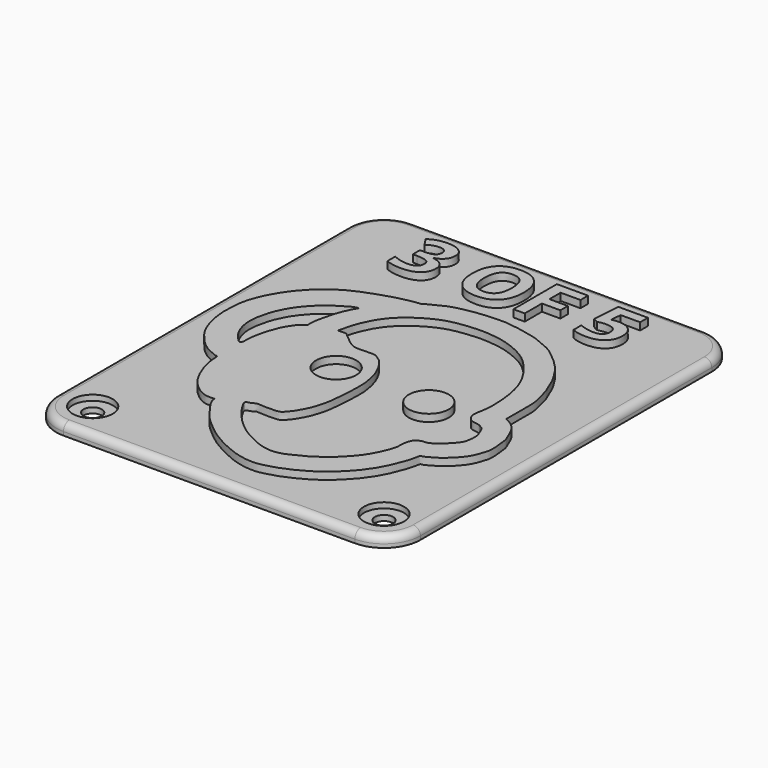
from build123d import *

# Parameters (mm, degrees)
F1_DEPTH     = 3
F2_R         = 5.5
F3_DEPTH     = 2
F4_R         = 2.5
F5_DEPTH     = 25
F4_R_2       = 5.5
F6_DEPTH     = 1.5
F7_R         = 2
F8_TEXT_SIZE = 20.8952981565
F9_DEPTH     = 2


# Not quite as in the source:
# - Text() gives the source's letters only with a copy of the font that has no kerning and outlines rounded to 1/6400 em; it was checked with that copy


with BuildPart() as f1:
    # F0 (on Top) → F1 (new body)
    with BuildSketch(Plane.XY):
        with BuildLine():
            Line((33.4852860868, 69.3044555187), (-46.5147139132, 69.3044555187))
            ThreePointArc((-46.5147139132, 69.3044555187), (-53.5857817251, 66.3755233306), (-56.5147139132, 59.3044555187))
            Line((-56.5147139132, 59.3044555187), (-56.5147139132, -40.6955444813))
            ThreePointArc((-56.5147139132, -40.6955444813), (-53.5857817251, -47.7666122931), (-46.5147139132, -50.6955444813))
            Line((-46.5147139132, -50.6955444813), (33.4852860868, -50.6955444813))
            ThreePointArc((33.4852860868, -50.6955444813), (40.5563538987, -47.7666122931), (43.4852860868, -40.6955444813))
            Line((43.4852860868, -40.6955444813), (43.4852860868, 59.3044555187))
            ThreePointArc((43.4852860868, 59.3044555187), (40.5563538987, 66.3755233306), (33.4852860868, 69.3044555187))
        make_face()
    extrude(amount=F1_DEPTH)

    # F2 (on face) → F3 (join)
    with BuildSketch(Plane.XY.offset(3)):
        with BuildLine():
            add(Edge.make_bspline(
                [(-18.6191648245, 37.6610159874), (-18.4103942017, 37.9016258723), (-16.7790980702, 38.6372652046), (-14.6637753752, 39.7765316628), (-13.2970537087, 40.3520065207), (-11.234009202, 40.9420295945), (-9.6324726991, 41.1696781496), (-8.0391436993, 41.5335651558), (-6.0169121605, 41.8153047571), (-4.3207068367, 41.9873935063), (-2.6143961302, 42.0419440702), (-0.9525336366, 42.1080518392), (1.0128601269, 42.1231970345), (2.1202521733, 41.9213075242), (4.0719475632, 41.6824185547), (5.8543562337, 41.3447673853), (8.2763433889, 40.8035747337), (10.1635651747, 40.353915966), (11.9937518037, 39.6067163832), (14.0226197173, 38.7871278462), (16.1856661814, 37.6734030141), (17.4924246856, 36.4788381138), (19.1253564081, 35.2746713919), (21.0525205789, 33.4368660129), (22.8143980711, 31.4334361407), (24.0610529234, 29.4392438038), (25.4962702164, 27.1113130015), (26.1960706131, 25.0093099567), (27.3364408686, 22.7329766681), (27.8343641487, 20.4595553566), (28.4512270226, 18.3747773676), (28.8543109039, 16.0260319825), (28.7482942364, 13.514319679), (28.7338146771, 10.334995111), (28.8639216748, 7.7618210354), (28.5892188921, 7.1456188181), (29.918494696, 6.6371361349), (30.7415769345, 6.048857602), (31.8218108898, 5.2284950474), (32.4881411718, 4.3144331607), (33.1106903749, 3.3497479147), (33.6641407706, 2.0109945661), (34.2180897974, 0.7680229197), (34.7699235136, -0.4925214664), (34.8393823017, -2.1248020855), (35.1159528786, -3.5786376005), (35.1890831283, -4.9707061488), (35.1986725747, -6.4306388091), (34.8113632413, -7.8018002545), (34.3648549572, -9.1685585465), (33.7006462016, -10.7925444113), (32.4786558474, -12.4867800792), (31.2093037355, -13.8794324624), (29.8228294921, -15.1123456384), (28.4481064283, -16.1979640059), (26.9010895599, -16.9942764857), (25.7560202386, -17.680414395), (25.0366948143, -17.6406684633), (24.9183175095, -18.4197855861), (24.4423119566, -20.5483511698), (23.952395564, -21.9587523538), (23.4131019879, -23.3338663207), (23.0363279372, -24.375840927), (22.2224307033, -26.1264489722), (21.2865086787, -27.8368274895), (20.1951867433, -29.4201151746), (18.9860862314, -31.1375710166), (17.3811137649, -32.8166180811), (15.7042926401, -34.5876163927), (13.5905636589, -36.4126926109), (11.1458686808, -38.0230479936), (8.6105659318, -39.4260561962), (6.3982038234, -40.4452898559), (3.9903626049, -41.4094407372), (1.5909701707, -42.0307219757), (-0.3244322342, -42.4472862511), (-3.0462389679, -42.3908445704), (-6.3739761828, -41.6795661098), (-9.0756360614, -40.5445583492), (-11.4999435367, -39.4334951706), (-14.0267237171, -38.0427328061), (-16.5231454021, -36.4228132711), (-19.2177237627, -34.0409247415), (-21.2287796931, -32.3535977287), (-22.9024936625, -30.0140416309), (-24.8830695481, -27.5285351284), (-25.7355527916, -25.7541093984), (-25.9204767707, -25.01094046), (-25.8155102433, -24.5585649767), (-26.3353607782, -24.6626985104), (-27.3937643857, -24.604343642), (-28.5385661833, -24.5736973327), (-29.8809336917, -24.0072466619), (-31.024992927, -23.3212546755), (-31.8421568409, -22.6244589116), (-32.6264406766, -22.0210900232), (-33.2706725903, -21.2034453928), (-34.1785245549, -20.2570422445), (-34.9266137095, -18.9229870195), (-35.7896187393, -17.4333249914), (-36.2943381796, -15.8618978444), (-36.9991849834, -14.3986458458), (-37.2894254224, -12.438873679), (-37.7598939793, -11.0391181733), (-37.7045092263, -8.5283318409), (-38.2366743053, -8.8861727805), (-39.6635712758, -8.1924450646), (-41.5724951076, -7.3876946804), (-42.9710227463, -6.2860034071), (-43.9844888849, -5.4484362874), (-44.8037531813, -4.4368938201), (-45.6767257624, -3.5007994876), (-46.4322786838, -2.5318099341), (-47.1103946136, -1.5496099297), (-47.7061145443, -0.4606324683), (-48.2107973432, 0.7930992035), (-48.6392724314, 1.9839832849), (-49.0279783093, 3.3434631602), (-49.3330366627, 4.6573318023), (-49.5371771144, 6.1611310797), (-49.8023387519, 8.0436742591), (-49.7003112223, 11.3243608595), (-49.3068712567, 14.7565338231), (-48.3770847842, 17.4395972901), (-47.3285912307, 19.9466829796), (-45.7808854328, 22.6784880165), (-43.6656800959, 25.7134230491), (-40.693893958, 28.6885478042), (-37.7553276892, 31.0585818166), (-34.4630210597, 33.006299034), (-30.4358052959, 34.5768091952), (-27.885204077, 35.4471267297), (-24.7077818652, 36.478027989), (-22.5428999706, 36.8875589665), (-20.6692139868, 37.2695632411), (-19.4417427743, 37.4537140356), (-18.7058739175, 37.3912967571), (-18.6926490505, 37.5763248036), (-18.6191648245, 37.6610159874)],
                knots=[0, 0, 0, 0, 0.0075309136, 0.0161573481, 0.0227755658, 0.0305866017, 0.0374962625, 0.0443748103, 0.0520858601, 0.059187183, 0.0661602068, 0.0732468426, 0.0807029903, 0.0865116291, 0.0939189243, 0.1013600191, 0.1098202957, 0.1173861998, 0.1248899916, 0.1329570033, 0.141339687, 0.1484834677, 0.1561072012, 0.1649609025, 0.1737747851, 0.1820999123, 0.190950056, 0.1990339225, 0.2075932835, 0.2158291335, 0.2237824706, 0.2320273243, 0.240587422, 0.2504983465, 0.259019864, 0.2627097894, 0.2686296425, 0.2743569361, 0.2805453142, 0.2862792826, 0.2920426192, 0.2985343623, 0.3048549054, 0.3111471155, 0.3180180172, 0.3246065295, 0.3309692703, 0.3374677437, 0.3438755839, 0.3503270105, 0.3574688719, 0.3652721138, 0.372717703, 0.380040523, 0.387197173, 0.3944005106, 0.4006027492, 0.4046360254, 0.4089424054, 0.4169607189, 0.4238009351, 0.4301881253, 0.4358992872, 0.443336293, 0.4509586354, 0.4584176636, 0.4662278316, 0.4744418396, 0.4828826611, 0.4918896868, 0.5011822198, 0.5103532814, 0.5187847155, 0.5274943105, 0.5359542485, 0.5434551126, 0.5522916039, 0.5623031135, 0.5715569002, 0.5803441106, 0.58944447, 0.5988462018, 0.6090545319, 0.6177946381, 0.626937173, 0.6366944691, 0.6441882891, 0.6488104973, 0.6518251884, 0.6551269878, 0.6607637291, 0.6666049253, 0.6730823753, 0.6793510941, 0.6849255641, 0.6902387749, 0.6957168326, 0.70186641, 0.7085624734, 0.71565831, 0.7225651249, 0.7294719417, 0.7368772857, 0.744012573, 0.751774301, 0.7546602097, 0.7612330205, 0.7692672645, 0.7764357762, 0.7825915376, 0.7887128919, 0.7948342416, 0.8008125502, 0.8066930468, 0.8127118393, 0.8189722105, 0.8250725008, 0.8314667434, 0.8377432378, 0.8442973391, 0.8517050547, 0.8615077536, 0.8716354601, 0.8806808608, 0.8895164581, 0.899036652, 0.9094568089, 0.9205341683, 0.9309948491, 0.9416272294, 0.9527577032, 0.9617764697, 0.9715282598, 0.9796501328, 0.9870668627, 0.9931898961, 0.9973492278, 1, 1, 1, 1], degree=3))
        make_face()
        with BuildLine():
            add(Edge.make_bspline(
                [(-38.0058884621, -0.5812315503), (-37.6090854426, -0.3774273349), (-37.7406822922, 2.2339313336), (-37.3711623907, 3.7843896417), (-37.054290198, 5.805401783), (-36.4511907485, 7.5657735533), (-35.7863149747, 9.5801695627), (-34.8925281411, 11.3432069096), (-33.5695259392, 13.1962010393), (-32.6566712986, 14.078855805), (-31.6524985285, 14.7306286565), (-31.8171843486, 15.1045410479), (-31.7501245212, 16.7053480485), (-31.478332639, 18.3041133796), (-30.9690870482, 20.3963769749), (-30.4969537954, 22.0647253275), (-30.1087344745, 23.3649568989), (-29.5363297053, 24.7107548242), (-28.9637690847, 25.9860533824), (-28.602542329, 26.7224913282), (-27.8451780879, 27.6326705597), (-28.7468525102, 27.5001263783), (-29.9683761689, 27.0621052555), (-31.2484707222, 26.1488736889), (-32.8753672069, 25.2858826755), (-34.0829626942, 24.2730936086), (-35.4207895878, 23.2420937515), (-36.7358234817, 22.0712007949), (-38.1958224081, 20.3551885046), (-39.6649709301, 18.4114272462), (-40.6002795558, 16.4851320334), (-41.3916501573, 14.8681126727), (-41.8868561359, 13.1908128068), (-42.2313507937, 11.57031163), (-42.5886797178, 10.157078484), (-42.6786597324, 8.2404148277), (-42.5759963307, 6.7415682502), (-42.2153347686, 5.1798783243), (-41.6860778269, 3.5343809817), (-40.5245375853, 1.585984149), (-39.5847971245, 0.5007867221), (-38.3271736854, -0.7462486486), (-38.0058884621, -0.5812315503)],
                knots=[0, 0, 0, 0, 0.0315996137, 0.0587260122, 0.0859538999, 0.1129907709, 0.1413306236, 0.1693430109, 0.1986512475, 0.2216392797, 0.2414291579, 0.2523814204, 0.2764712507, 0.3024633699, 0.3312084147, 0.3571365343, 0.3798507092, 0.4037305378, 0.4266685212, 0.4456738987, 0.4633706866, 0.4775024547, 0.5004991818, 0.525334492, 0.551894368, 0.5766039012, 0.6018897439, 0.6278991303, 0.6573875722, 0.6882127238, 0.7169035956, 0.7431609544, 0.7690890029, 0.794183922, 0.8180148, 0.8450104008, 0.8692265117, 0.8936965249, 0.9197979433, 0.9487499704, 0.974414285, 1, 1, 1, 1], degree=3))
        make_face(mode=Mode.SUBTRACT)
        with Locations((-14.579073526, 2.9678073493)):
            Circle(F2_R, mode=Mode.SUBTRACT)
        with BuildLine():
            add(Edge.make_bspline(
                [(26.1008664966, 1.2549897656), (26.2928987951, 1.1656873111), (26.6964760721, 0.9779096942), (27.3683049725, 0.5337475949), (27.8014603626, -0.35845667), (28.1392882182, -1.0393573393), (28.4250008951, -1.7666657733), (28.7772740298, -2.9138156663), (28.804871187, -4.2022706979), (28.6020847246, -5.6518966997), (28.2775658027, -6.8563748795), (27.4326796061, -8.0439049534), (26.4420205117, -9.1672069315), (24.9107731491, -10.454736586), (23.9147678264, -11.2637788499), (22.6044329122, -12.1541535735), (21.2664242249, -12.0478940652), (20.4618789241, -12.3713253406), (19.5960482955, -12.8341187078), (19.1056099781, -13.6445877873), (18.742577739, -14.9014126996), (18.5833338196, -16.308245582), (18.6956398455, -17.5783829814), (18.0150457409, -19.6557956816), (17.1397510563, -21.6691745731), (16.115950725, -23.7092902312), (14.7452402396, -25.6827628343), (13.3829900637, -27.2074203377), (12.1330645973, -28.5821514887), (10.5308526761, -30.0685235538), (9.0765905709, -31.1053628256), (7.3253353057, -32.4298147228), (5.5726928858, -33.407876634), (2.9036342484, -34.6752714482), (1.7989995119, -35.2447034015), (0.2625602707, -35.6817813116), (-0.6389409084, -35.7890471044), (-2.0871349328, -35.877007594), (-3.8497452527, -35.5162376915), (-5.222457709, -35.0816197537), (-6.8221021482, -34.4501167282), (-8.4763307857, -33.5402713175), (-9.6302218537, -32.968880321), (-10.8790005442, -32.2277682746), (-12.0019794322, -31.4372092635), (-12.9644892688, -30.6688877688), (-13.9755730142, -29.6855780121), (-14.7880117168, -29.0074116251), (-15.6447686252, -28.1262570516), (-16.3360017365, -27.268464228), (-17.1774534348, -26.3070483764), (-17.8078869532, -25.4449799373), (-18.481499733, -24.6125230577), (-18.9894242484, -23.7845906216), (-19.4860111205, -22.8717611575), (-19.8388559456, -22.2710179536), (-19.9048971425, -21.563110618), (-18.8815847964, -21.2771650947), (-18.3039836749, -21.1290999033), (-17.5299430613, -20.5392938554), (-16.7443590677, -20.7296600024), (-11.6236967061, -20.8700323771), (-10.6837289364, -20.2035585312), (-10.0595009134, -19.4857888595), (-9.1855924768, -18.4285627789), (-8.54418321, -17.3503474591), (-7.6747900037, -15.8205265417), (-7.0231596712, -14.351105049), (-6.5858424855, -12.8180238092), (-6.1056784276, -11.210482169), (-5.7031118195, -8.9522904228), (-5.5245802408, -5.7526252941), (-5.2997192835, -3.1041005432), (-5.2389990659, -0.0071802216), (-5.3208156943, 1.4791379717), (-5.6404910304, 3.3489073836), (-6.0644365636, 5.0374394573), (-6.4445575041, 6.305566795), (-7.0058328991, 7.4315033704), (-7.4567235246, 8.4571218702), (-7.8416896889, 9.0668786743), (-8.3018280382, 9.8511130455), (-8.7589041464, 10.4376252677), (-9.2006522413, 11.0101977678), (-9.8406836062, 11.6509719694), (-10.763933157, 12.242007809), (-11.4899920131, 12.6906880936), (-12.2487513325, 12.9617424798), (-14.3613578729, 12.8272603912), (-15.7496441884, 12.8251488381), (-17.2050199699, 12.7619968464), (-18.3214726369, 13.244892088), (-19.4165259237, 13.8766007999), (-20.3209782258, 14.6408246043), (-21.023021958, 15.1948783171), (-21.7378218012, 15.8131392854), (-22.2637216579, 16.2352537848), (-22.7816344022, 16.7217796073), (-23.0545999832, 16.7391538664), (-23.633456708, 16.7266977055), (-24.1478196183, 16.7192518065), (-24.5020069236, 16.7230805303), (-24.8687583036, 16.6790353571), (-25.0056890792, 16.7532505515), (-25.065490976, 16.7856626213)],
                knots=[0, 0, 0, 0, 0.0069852497, 0.0146819314, 0.0232537871, 0.030808328, 0.0384124369, 0.0478279818, 0.0577533282, 0.0682054513, 0.0778667647, 0.0881384633, 0.0989228018, 0.1110874431, 0.1211005813, 0.1317687759, 0.1415936754, 0.1496181769, 0.1579979053, 0.166289783, 0.1762128955, 0.186468199, 0.1961996569, 0.2088500225, 0.2218544675, 0.2349611313, 0.248411856, 0.2607660116, 0.2726212999, 0.2853371524, 0.2970449745, 0.3096528258, 0.3223082686, 0.3370210916, 0.3469985445, 0.3576176679, 0.3659605218, 0.3762720077, 0.3879312736, 0.3983551213, 0.4097473692, 0.4216535998, 0.4315400734, 0.4419180766, 0.4520777768, 0.4617615717, 0.4719835241, 0.4809868969, 0.4904812275, 0.4996776368, 0.5094331744, 0.5184583815, 0.5273540811, 0.5359798129, 0.5448015969, 0.5521029504, 0.5585464321, 0.5668719463, 0.5739565372, 0.581807992, 0.589843085, 0.6092713546, 0.6185326035, 0.6266765048, 0.6367584326, 0.6465963096, 0.6580409486, 0.6691161436, 0.6799667249, 0.6910940016, 0.7042496242, 0.7197264468, 0.7342582186, 0.7492921819, 0.7599675109, 0.7717718945, 0.7833001624, 0.7932397434, 0.8029942498, 0.8120924964, 0.8194884005, 0.8276856603, 0.8351893613, 0.842482553, 0.8507424198, 0.8598828257, 0.8677483522, 0.8754313848, 0.8879028672, 0.8984945059, 0.9087094944, 0.9182048029, 0.9279759377, 0.9373793148, 0.9456410344, 0.9539664127, 0.9613182768, 0.9683568791, 0.9727834066, 0.9793272295, 0.9856413964, 0.9908446381, 0.9960003839, 1, 1, 1, 1], degree=3))
            add(Edge.make_bspline(
                [(-25.065490976, 16.7856626213), (-24.7558959843, 18.1691471419), (-24.1022558698, 21.0901053034), (-21.8658687578, 25.9232720017), (-18.5384939524, 29.9131247419), (-13.5554986887, 33.273654491), (-8.917318544, 35.1618815245), (-3.7364368359, 35.7548445037), (-0.0083563057, 35.9514384456), (5.6240966531, 35.3461987753), (10.607407865, 33.3133844835), (14.171452126, 31.1673119591), (17.9214747103, 26.9190188236), (20.6977140843, 22.4145841063), (22.0168186297, 17.6172119697), (22.5488334108, 13.429796195), (22.6716420215, 9.8339043682), (22.3717474393, 6.7575340001), (21.6179450683, 3.8501564166), (23.5244445313, 1.3505182234), (25.1325760037, 1.6951217549), (26.1008664966, 1.2549897656)],
                knots=[0, 0, 0, 0, 0.0526736814, 0.1102669532, 0.1677376719, 0.2289088422, 0.2856783657, 0.3421651676, 0.3911077782, 0.4505991711, 0.5089139673, 0.5599984994, 0.619312872, 0.6775862208, 0.7334100044, 0.7851630524, 0.8326643854, 0.8770150871, 0.9197823607, 0.9597160451, 1, 1, 1, 1], degree=3))
        make_face(mode=Mode.SUBTRACT)
        with Locations((10.8706516725, 2.9678073493)):
            Circle(F2_R)
    extrude(amount=F3_DEPTH)

    # F4 (on face) → F5 (cut)
    with BuildSketch(Plane.XY.offset(3)):
        with Locations((-46.5147139132, -40.6955444813)):
            Circle(F4_R)
        with Locations((33.4852860868, -40.6955444813)):
            Circle(F4_R)
    extrude(amount=-F5_DEPTH, mode=Mode.SUBTRACT)

    # F4 (on face) → F6 (cut)
    with BuildSketch(Plane.XY.offset(3)):
        with Locations((-46.5147139132, -40.6955444813)):
            Circle(F4_R_2)
        with Locations((-46.5147139132, -40.6955444813)):
            Circle(F4_R, mode=Mode.SUBTRACT)
        with Locations((33.4852860868, -40.6955444813)):
            Circle(F4_R_2)
        with Locations((33.4852860868, -40.6955444813)):
            Circle(F4_R, mode=Mode.SUBTRACT)
    extrude(amount=-F6_DEPTH, mode=Mode.SUBTRACT)

    # F7
    f7_edges = [f1.edges().sort_by_distance(p)[0] for p in [
        (-6.514714, -50.695544, 3),
    ]]
    fillet(f7_edges, radius=F7_R)

    # F8 (on face) → F9 (join)
    with BuildSketch(Plane.XY.offset(3)):
        with Locations((-37.7322882414, 47.9189679027)):
            Text('3 OF 5', F8_TEXT_SIZE, font='Open Sans', font_style=FontStyle.BOLD, text_align=(TextAlign.LEFT, TextAlign.BOTTOM))
    extrude(amount=F9_DEPTH)


solid = f1.part
